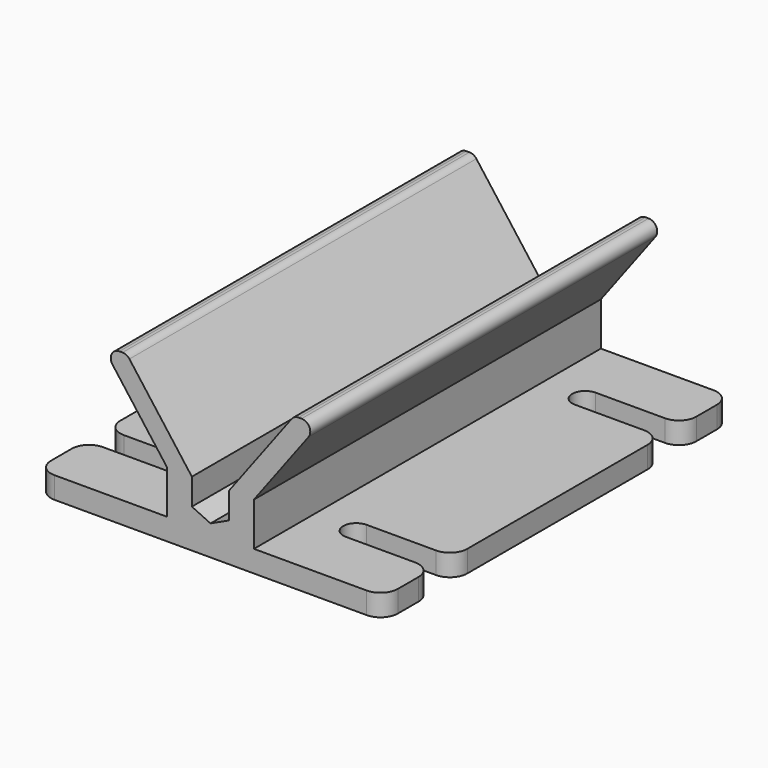
from build123d import *

# Parameters (mm, degrees)
F0_W     = 101.6
F0_H     = 44.45
F1_DEPTH = 63.5
F3_DEPTH = 127.001
F5_DEPTH = 127.001
F6_R     = 2.54
F8_DEPTH = 6.35
F9_R     = 5.08


# Not quite as in the source:
# - a pattern or mirror of a feature is missing from the dataset's text; its kind, count and spacing are read off the source's solid


with BuildPart() as f1:
    # F0 (on Front) → F1 (new body, symmetric)
    with BuildSketch(Plane.XZ):
        Rectangle(F0_W, F0_H)
    extrude(amount=F1_DEPTH, both=True)

    # F2 (on face) → F3 (cut, through all)
    with BuildSketch(Plane.XZ.offset(63.5)):
        Polygon((-50.8, -15.875), (-12.7, -15.875), (-12.7, -3.175), (-31.75, 22.225), (-50.8, 22.225), align=None)
    f3 = extrude(amount=-F3_DEPTH, mode=Mode.SUBTRACT)

    # F3_copies: F3 across plane
    add(f3.mirror(Plane(origin=(0, 0, 0), x_dir=(0, 0, 1), z_dir=(1, 0, 0))), mode=Mode.SUBTRACT)

    # F4 (on face) → F5 (cut, through all)
    with BuildSketch(Plane.XZ.offset(63.5)):
        Polygon((24.511, 22.225), (-24.511, 22.225), (-5.461, -3.175), (-5.461, -10.8996083293), (0, -13.4461144505), (5.461, -10.8996083293), (5.461, -3.175), align=None)
    extrude(amount=-F5_DEPTH, mode=Mode.SUBTRACT)

    # F6
    f6_edges = [f1.edges().sort_by_distance(p)[0] for p in [
        (-31.75, 0, 22.225),
        (-24.511, 0, 22.225),
        (24.511, 0, 22.225),
        (31.75, 0, 22.225),
    ]]
    fillet(f6_edges, radius=F6_R)

    # F7 (on face) → F8 (cut, through all)
    with BuildSketch(Plane(origin=(0, 0, -22.225), x_dir=(1, 0, 0), z_dir=(0, 0, -1))):
        with BuildLine():
            Line((-25.4, 45.72), (-50.8, 45.72))
            Line((-50.8, 45.72), (-50.8, 38.1))
            Line((-50.8, 38.1), (-25.4, 38.1))
            ThreePointArc((-25.4, 38.1), (-21.59, 41.91), (-25.4, 45.72))
        make_face()
        with BuildLine():
            Line((-25.4, -38.1), (-50.8, -38.1))
            Line((-50.8, -38.1), (-50.8, -45.72))
            Line((-50.8, -45.72), (-25.4, -45.72))
            ThreePointArc((-25.4, -45.72), (-21.59, -41.91), (-25.4, -38.1))
        make_face()
    f8 = extrude(amount=-F8_DEPTH, mode=Mode.SUBTRACT)

    # F8_copies: F8 across plane
    add(f8.mirror(Plane(origin=(0, 0, 0), x_dir=(0, 0, 1), z_dir=(1, 0, 0))), mode=Mode.SUBTRACT)

    # F9
    f9_edges = [f1.edges().sort_by_distance(p)[0] for p in [
        (-50.8, -63.5, -19.05),
        (-50.8, 63.5, -19.05),
        (50.8, -63.5, -19.05),
        (50.8, 63.5, -19.05),
        (-50.8, -45.72, -19.05),
        (-50.8, 38.1, -19.05),
        (-50.8, 45.72, -19.05),
        (-50.8, -38.1, -19.05),
        (50.8, 45.72, -19.05),
        (50.8, -45.72, -19.05),
        (50.8, -38.1, -19.05),
        (50.8, 38.1, -19.05),
    ]]
    fillet(f9_edges, radius=F9_R)


solid = f1.part
